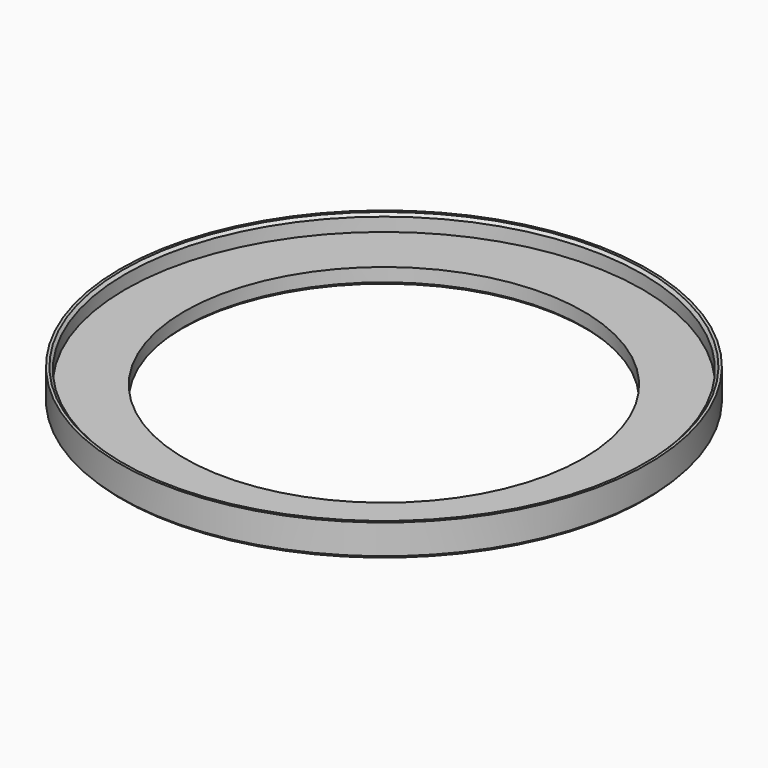
from build123d import *

# Parameters (mm, degrees)
F2_SIZE      = 0.5
F3_TEXT_SIZE = 8.3333333333
F1_FACE1_R   = 49
F1_FACE1_R_2 = 48.5
F4_DEPTH     = 1


# Not quite as in the source:
# - a feature names something its author has since deleted; it is built from what else it names
# - Text() gives the source's letters only with a copy of the font that has no kerning and outlines rounded to 1/6400 em; it was checked with that copy


with BuildPart() as f1:
    # F0 (on Front) → F1 (revolve)
    with BuildSketch(Plane.XZ):
        Polygon((-48, 6), (-49, 6), (-49, 0), (-37, 0), (-37, 3), (-48, 3), align=None)
    revolve(axis=Axis((0, 0, 17.5639875233), (0, 0, -1)))

    # F2
    f2_edges = [f1.edges().sort_by_distance(p)[0] for p in [
        (49, 0, 0),
        (37, 0, 0),
        (48, 0, 6),
    ]]
    chamfer(f2_edges, length=F2_SIZE)

    # F3 (on face) + F1_face1 (on face) → F4 (cut)
    with BuildSketch(Plane(origin=(0, 0, 0), x_dir=(1, 0, 0), z_dir=(0, 0, -1))):
        with Locations((-12.4479166667, 39.5)):
            Text('61mm', F3_TEXT_SIZE, font='Open Sans', text_align=(TextAlign.LEFT, TextAlign.BOTTOM))
    with BuildSketch(Plane.XY.offset(6)):
        Circle(F1_FACE1_R)
        Circle(F1_FACE1_R_2, mode=Mode.SUBTRACT)
    extrude(amount=-F4_DEPTH, dir=(0, 0, -1), mode=Mode.SUBTRACT)


solid = f1.part
